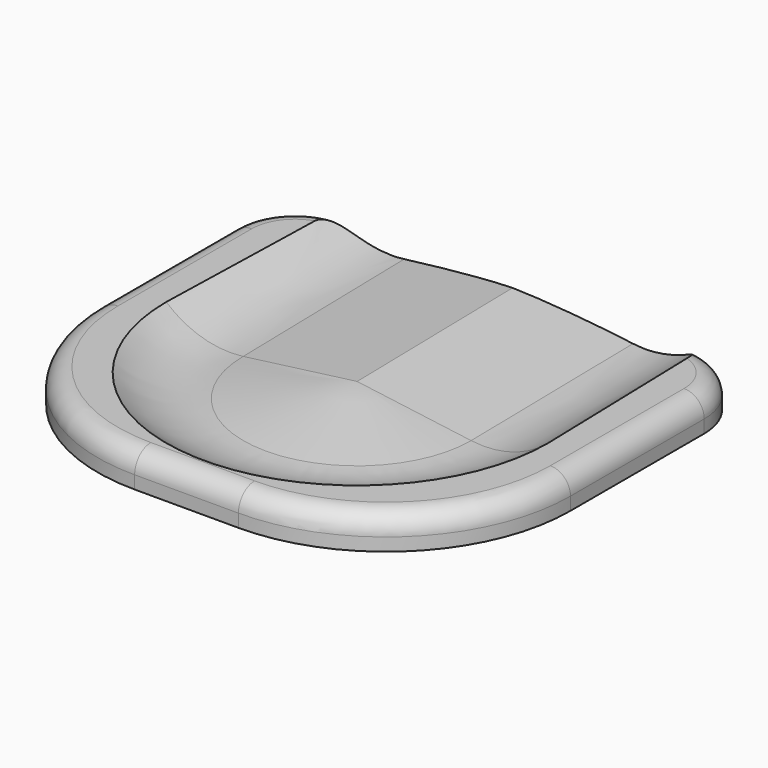
from build123d import *

# Parameters (mm, degrees)
F0_W     = 520.7
F0_H     = 457.2
F1_DEPTH = 36.5125
F2_R     = 203.2
F3_R     = 69.85
F4_R     = 22.225
F6_DEPTH = 222.25
F6_TAPER = -1
F8_ANGLE = 180


# Not quite as in the source:
# - a feature names something its author has since deleted; it is built from what else it names


with BuildPart() as f1:
    # F0 (on Top) → F1 (new body)
    with BuildSketch(Plane.XY):
        Rectangle(F0_W, F0_H)
    extrude(amount=F1_DEPTH)

    # F2
    f2_edges = [f1.edges().sort_by_distance(p)[0] for p in [
        (-260.35, -228.6, 18.25625),
        (260.35, -228.6, 18.25625),
    ]]
    fillet(f2_edges, radius=F2_R)

    # F3
    f3_edges = [f1.edges().sort_by_distance(p)[0] for p in [
        (260.35, 228.6, 18.25625),
        (-260.35, 228.6, 18.25625),
    ]]
    fillet(f3_edges, radius=F3_R)

    # F4
    f4_edges = [f1.edges().sort_by_distance(p)[0] for p in [
        (0, 228.6, 36.5125),
    ]]
    fillet(f4_edges, radius=F4_R)

    # F5 (on face) → F6 (cut)
    with BuildSketch(Plane(origin=(0, 228.6, 0), x_dir=(-1, 0, 0), z_dir=(0, 1, 0))):
        with BuildLine():
            Line((0, 181.2540946981), (-105.1541626057, 217.9785540242))
            ThreePointArc((-105.1541626057, 217.9785540242), (-243.9245415433, 129.7884295676), (-126.0241182101, 15.1838646496))
            Line((-126.0241182101, 15.1838646496), (0, 31.7752545682))
            Line((0, 31.7752545682), (126.0241182101, 15.1838646496))
            ThreePointArc((126.0241182101, 15.1838646496), (243.9245415433, 129.7884295676), (105.1541626057, 217.9785540242))
            Line((105.1541626057, 217.9785540242), (0, 181.2540946981))
        make_face()
    extrude(amount=-F6_DEPTH, taper=F6_TAPER, mode=Mode.SUBTRACT)

    # F7 (on face) → F8 (revolve, cut)
    with BuildSketch(Plane(origin=(0, 6.35, 0), x_dir=(-1, 0, 0), z_dir=(0, 1, 0))):
        with BuildLine():
            Line((0, 36.5125), (-210.3489459995, 36.5125))
            ThreePointArc((-210.3489459995, 36.5125), (-170.6122176221, 14.8981545045), (-125.5177564428, 11.3376651729))
            Line((-125.5177564428, 11.3376651729), (0, 27.8623913002))
            Line((0, 27.8623913002), (0, 36.5125))
        make_face()
    revolve(axis=Axis((0, 6.35, 32.1874456501), (0, 0, -1)), revolution_arc=F8_ANGLE, mode=Mode.SUBTRACT)


solid = f1.part
